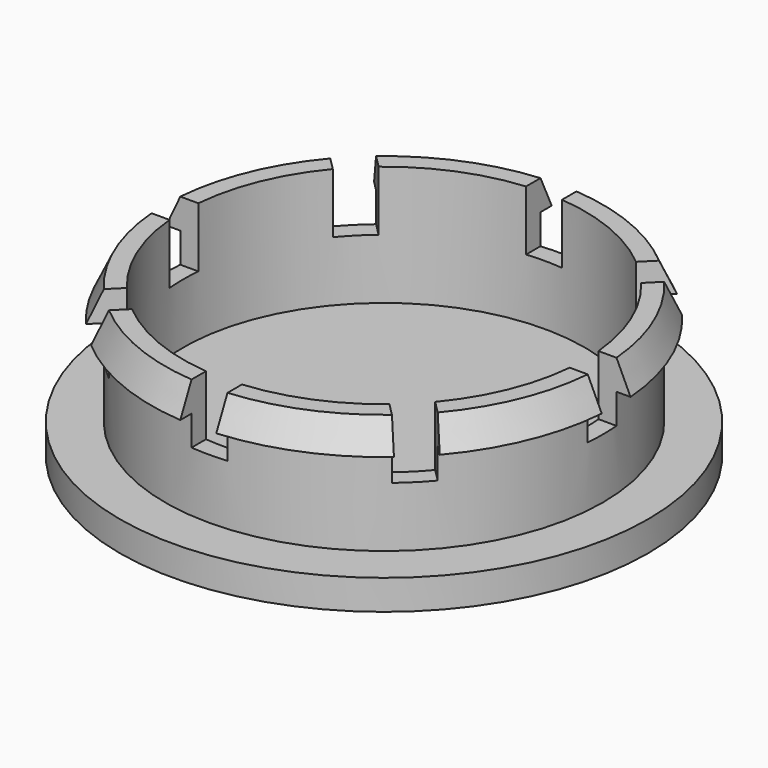
from build123d import *

# Parameters (mm, degrees)
F0_R      = 36.5
F0_R_2    = 33.5
F1_DEPTH  = 20
F2_R      = 36.5
F3_DEPTH  = 5
F3_TAPER  = -25
F4_R      = 33.5
F5_DEPTH  = 25
F6_R      = 44.05
F7_DEPTH  = 5
F10_DEPTH = 25


# Not quite as in the source:
# - a pattern or mirror of a feature is missing from the dataset's text; its kind, count and spacing are read off the source's solid


with BuildPart() as f1:
    # F0 (on Top) → F1 (new body)
    with BuildSketch(Plane.XY):
        Circle(F0_R)
        Circle(F0_R_2, mode=Mode.SUBTRACT)
    extrude(amount=F1_DEPTH)

    # F2 (on face) → F3 (join)
    with BuildSketch(Plane.XY.offset(20)):
        Circle(F2_R)
    extrude(amount=-F3_DEPTH, taper=F3_TAPER)

    # F4 (on face) → F5 (cut)
    with BuildSketch(Plane(origin=(0, 0, 15), x_dir=(1, 0, 0), z_dir=(0, 0, -1))):
        Circle(F4_R)
    extrude(amount=-F5_DEPTH, mode=Mode.SUBTRACT)

    # F6 (on face) → F7 (join)
    with BuildSketch(Plane(origin=(0, 0, 0), x_dir=(1, 0, 0), z_dir=(0, 0, -1))):
        Circle(F6_R)
    extrude(amount=F7_DEPTH)

    # F9 (on mid) → F10 (cut)
    with BuildSketch(Plane.XY.offset(10)):
        with BuildLine():
            Line((35.05, 3), (3, 3))
            Line((3, 3), (3, 35.05))
            Line((3, 35.05), (3, 38.3829389182))
            ThreePointArc((3, 38.3829389182), (0, 38.5), (-3, 38.3829389182))
            Line((-3, 38.3829389182), (-3, 35.05))
            Line((-3, 35.05), (-3, 3))
            Line((-3, 3), (-38.3829389182, 3))
            Line((-38.3829389182, 3), (-61.3953992724, 3))
            Line((-61.3953992724, 3), (-61.3953992724, -3))
            Line((-61.3953992724, -3), (-3, -3))
            Line((-3, -3), (-3, -40.2699470416))
            Line((-3, -40.2699470416), (-3, -53.7798181176))
            Line((-3, -53.7798181176), (3, -53.7798181176))
            Line((3, -53.7798181176), (3, -40.2699470416))
            Line((3, -40.2699470416), (3, -29.05))
            Line((3, -29.05), (3, -3))
            Line((3, -3), (61.3953992724, -3))
            Line((61.3953992724, -3), (61.3953992724, 3))
            Line((61.3953992724, 3), (38.3829389182, 3))
            Line((38.3829389182, 3), (35.05, 3))
        make_face()
        with BuildLine():
            ThreePointArc((-3, 38.3829389182), (0, 38.5), (3, 38.3829389182))
            Line((3, 38.3829389182), (3, 40.2699470416))
            Line((3, 40.2699470416), (3, 53.7798181176))
            Line((3, 53.7798181176), (-3, 53.7798181176))
            Line((-3, 53.7798181176), (-3, 40.2699470416))
            Line((-3, 40.2699470416), (-3, 38.3829389182))
        make_face()
    f10 = extrude(amount=F10_DEPTH, mode=Mode.SUBTRACT)

    # F10_copies: F10 across plane
    add(f10.mirror(Plane(origin=(0, 0, 0), x_dir=(0.3826834319, -0.9238795327, 0), z_dir=(-0.9238795327, -0.3826834319, 6e-10))), mode=Mode.SUBTRACT)


solid = f1.part
